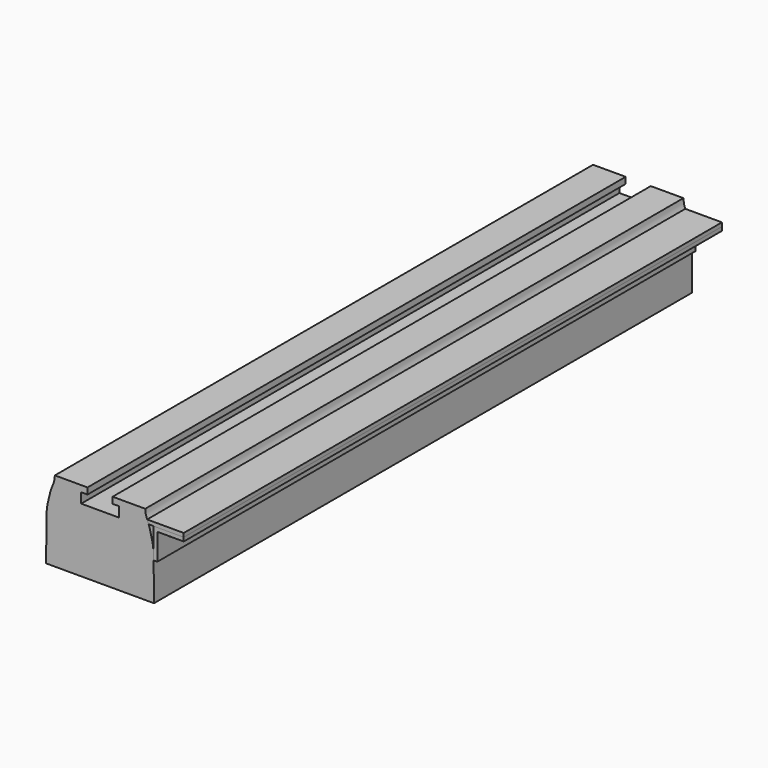
from build123d import *

# Parameters (mm, degrees)
F1_DEPTH    = 1701.8
F2_T        = 12.7
F2_T3_DEPTH = 1727.2
F3_DEPTH    = 1701.8
F4_DEPTH    = 1701.8
F5_R        = 4.7625
F6_DEPTH    = 76.2
F7_R        = 4.7625
F8_DEPTH    = 38.1
F9_DEPTH    = 7.9502


# Not quite as in the source:
# - a shell that OpenCascade refuses in one call is made with other operations: the cavity is built on its own and cut out


with BuildPart() as f1:
    # F0 (on Front) → F1 (new body)
    with BuildSketch(Plane.XZ):
        with BuildLine():
            add(Edge.make_bspline(
                [(22.225, 203.2), (21.8642991609, 198.9436880719), (21.1344297725, 190.3311442484), (16.2062788464, 177.7659442367), (11.0503834246, 165.2296560586), (8.3197375625, 152.3981513973), (4.8439366382, 139.6834435797), (2.2250256216, 127.2785692933), (1.2286177198, 113.4648940726), (1.0135363596, 99.4317737399), (0.4306333737, 42.2467726736), (0, 0)],
                knots=[0, 0, 0, 0, 0.0918377354, 0.1858314274, 0.2803034725, 0.3731848965, 0.4660441611, 0.5583399226, 0.6499464605, 0.7413896645, 1, 1, 1, 1], degree=3))
            Line((0, 0), (136.525, 0))
            Line((136.525, 0), (273.05, 0))
            add(Edge.make_bspline(
                [(272.0569275252, 95.25), (272.2812266122, 75.4195947963), (272.6656133061, 37.7097973982), (273.05, 0)],
                knots=[0.7691624061, 0.7691624061, 0.7691624061, 0.7691624061, 1, 1, 1, 1], degree=3))
            add(Edge.make_bspline(
                [(259.3917865325, 171.45), (260.1994606069, 169.3420370399), (262.4611803115, 163.060734298), (264.7302624375, 152.3981513973), (268.2060633618, 139.6834435797), (270.8249743784, 127.2785692933), (271.8213822802, 113.4648940726), (271.9240494417, 106.7663097297), (272.0299414505, 97.6358536592), (272.0569275252, 95.25)],
                knots=[0.2331960594, 0.2331960594, 0.2331960594, 0.2331960594, 0.2803034725, 0.3731848965, 0.4660441611, 0.5583399226, 0.6499464605, 0.7413896645, 0.7691624061, 0.7691624061, 0.7691624061, 0.7691624061], degree=3))
            Line((259.3917865325, 171.45), (257.0350068766, 177.3899913101))
            add(Edge.make_bspline(
                [(255.612601505, 180.975), (256.0230639926, 179.9152345168), (256.500145149, 178.7204324571), (256.980044358, 177.5266491388), (257.0350068766, 177.3899913101)],
                knots=[0.1621762876, 0.1621762876, 0.1621762876, 0.1621762876, 0.1858314274, 0.1888896754, 0.1888896754, 0.1888896754, 0.1888896754], degree=3))
            add(Edge.make_bspline(
                [(250.825, 203.2), (251.1857008391, 198.9436880719), (251.822662571, 191.4274654202), (254.3920914035, 184.1262123929), (255.612601505, 180.975)],
                knots=[0, 0, 0, 0, 0.0918377354, 0.1621762876, 0.1621762876, 0.1621762876, 0.1621762876], degree=3))
            Line((250.825, 203.2), (168.275, 203.2))
            Line((168.275, 203.2), (168.275, 187.325))
            Line((168.275, 187.325), (184.15, 187.325))
            Line((184.15, 187.325), (184.15, 161.925))
            Line((184.15, 161.925), (136.525, 161.925))
            Line((136.525, 161.925), (88.9, 161.925))
            Line((88.9, 161.925), (88.9, 187.325))
            Line((88.9, 187.325), (104.775, 187.325))
            Line((104.775, 187.325), (104.775, 203.2))
            Line((104.775, 203.2), (22.225, 203.2))
        make_face()
    extrude(amount=F1_DEPTH)

    # F2: shell of thickness 12.7, made by hand


with BuildPart() as f2_core1:
    # F2_t2: copy of F1
    add(f1.part)

    # the walls: a layer under each face that stays
    f2_faces = [f2_core1.faces().sort_by_distance(p)[0] for p in [
        (3.9234483512, -850.9, 135.090556138),
        (136.525, -1701.8, 101.6),
        (104.775, -850.9, 195.2625),
        (96.8375, -850.9, 187.325),
        (88.9, -850.9, 174.625),
        (136.525, -850.9, 161.925),
        (184.15, -850.9, 174.625),
        (176.2125, -850.9, 187.325),
        (168.275, -850.9, 195.2625),
        (209.55, -850.9, 203.2),
        (252.207010635, -850.9, 191.9731178888),
        (256.3176106399, -850.9, 179.181336214),
        (258.2133967045, -850.9, 174.4199956551),
        (269.1606720318, -850.9, 134.9300335195),
        (272.49343091, -850.9, 54.3297720729),
        (136.525, 0, 101.6),
        (63.5, -850.9, 203.2),
    ]]
    thicken(f2_faces, amount=-F2_T, mode=Mode.SUBTRACT)

    # F2_s4 → F2_t3 (cut)
    with BuildSketch(Plane.XZ.offset(-12.7)):
        Polygon((89.027, 187.198), (88.9, 200.025), (76.2, 200.025), (76.2, 187.325), align=None)
        Polygon((89.027, 162.052), (76.2, 161.925), (76.2, 149.225), (88.9, 149.225), align=None)
        Polygon((184.023, 162.052), (184.15, 149.225), (196.85, 149.225), (196.85, 161.925), align=None)
        Polygon((184.023, 187.198), (196.85, 187.325), (196.85, 200.025), (184.15, 200.025), align=None)
    extrude(amount=F2_T3_DEPTH, mode=Mode.SUBTRACT)


with BuildPart() as f1_1:
    add(f1.part)

    # what is left inside the walls is the cavity
    f2_cavity = [f2_core1.part.solids().sort_by_distance(p)[0] for p in [
        (136.525, -1130.3, 0.127),
    ]]
    add(f2_cavity, mode=Mode.SUBTRACT)


with BuildPart() as f3:
    # F0 (on Front) → F3 (new body)
    with BuildSketch(Plane.XZ):
        with BuildLine():
            add(Edge.make_bspline(
                [(257.0350068766, 177.3899913101), (257.831276655, 175.410160296), (258.6321371426, 173.4326224799), (259.3917865325, 171.45)],
                knots=[0.1888896754, 0.1888896754, 0.1888896754, 0.1888896754, 0.2331960594, 0.2331960594, 0.2331960594, 0.2331960594], degree=3))
            Line((259.3917865325, 171.45), (272.0569275252, 171.45))
            Line((272.0569275252, 171.45), (348.2569275252, 171.45))
            Line((348.2569275252, 171.45), (348.2569275252, 180.975))
            Line((348.2569275252, 180.975), (255.612601505, 180.975))
            Line((255.612601505, 180.975), (257.0350068766, 177.3899913101))
        make_face()
    extrude(amount=F3_DEPTH)


with BuildPart() as f4:
    # F0 (on Front) → F4 (new body)
    with BuildSketch(Plane.XZ):
        Polygon((272.0569275252, 171.45), (272.0569275252, 95.25), (281.5819275252, 95.25), (281.5819275252, 161.925), (348.2569275252, 161.925), (348.2569275252, 171.45), align=None)
    extrude(amount=F4_DEPTH)


with BuildPart() as f6_tool:
    # F5 (on face) → F6 (new body)
    with BuildSketch(Plane.YZ.offset(281.5819275252)):
        with Locations((-1663.7, 146.0500000011)):
            Circle(F5_R)
        with Locations((-1392.7666666667, 146.0500000011)):
            Circle(F5_R)
        with Locations((-1121.8333333333, 146.0500000011)):
            Circle(F5_R)
        with Locations((-850.9, 146.0500000011)):
            Circle(F5_R)
        with Locations((-579.9666666667, 146.0500000011)):
            Circle(F5_R)
        with Locations((-309.0333333333, 146.0500000011)):
            Circle(F5_R)
        with Locations((-38.1, 146.0500000011)):
            Circle(F5_R)
    extrude(amount=-F6_DEPTH)


with BuildPart() as f1_2:
    add(f1_1.part)

    # F6: cut by f6_tool
    add(f6_tool.part, mode=Mode.SUBTRACT)


with BuildPart() as f4_1:
    add(f4.part)

    # F6: cut by f6_tool
    add(f6_tool.part, mode=Mode.SUBTRACT)


with BuildPart() as f8:
    # F7 (on face) → F8 (new body)
    with BuildSketch(Plane.YZ.offset(281.5819275252)):
        with Locations((-1663.7, 146.0500000011)):
            Circle(F7_R)
    extrude(amount=-F8_DEPTH)

    # F7 (on face) + F5 (on face) → F9 (join)
    with BuildSketch(Plane.YZ.offset(281.5819275252)):
        Polygon((-1667.8244459855, 138.9062500011), (-1659.5755540145, 138.9062500011), (-1655.451108029, 146.0500000011), (-1659.5755540145, 153.1937500011), (-1667.8244459855, 153.1937500011), (-1671.948891971, 146.0500000011), align=None)
        with Locations((-1663.7, 146.0500000011)):
            Circle(F7_R, mode=Mode.SUBTRACT)
    with BuildSketch(Plane.YZ.offset(281.5819275252)):
        with Locations((-1663.7, 146.0500000011)):
            Circle(F5_R)
    extrude(amount=F9_DEPTH)


with BuildPart() as f8b:
    # F7 (on face) → F8, piece 2 (new body)
    with BuildSketch(Plane.YZ.offset(281.5819275252)):
        with Locations((-1392.7666666667, 146.0500000011)):
            Circle(F7_R)
    extrude(amount=-F8_DEPTH)

    # F7 (on face) + F5 (on face) → F9, piece 2 (join)
    with BuildSketch(Plane.YZ.offset(281.5819275252)):
        Polygon((-1384.5177746956, 146.0500000011), (-1388.6422206811, 153.1937500011), (-1396.8911126522, 153.1937500011), (-1401.0155586377, 146.0500000011), (-1396.8911126522, 138.9062500011), (-1388.6422206811, 138.9062500011), align=None)
        with Locations((-1392.7666666667, 146.0500000011)):
            Circle(F7_R, mode=Mode.SUBTRACT)
    with BuildSketch(Plane.YZ.offset(281.5819275252)):
        with Locations((-1392.7666666667, 146.0500000011)):
            Circle(F5_R)
    extrude(amount=F9_DEPTH)


with BuildPart() as f8c:
    # F7 (on face) → F8, piece 3 (new body)
    with BuildSketch(Plane.YZ.offset(281.5819275252)):
        with Locations((-1121.8333333333, 146.0500000011)):
            Circle(F7_R)
    extrude(amount=-F8_DEPTH)

    # F7 (on face) + F5 (on face) → F9, piece 3 (join)
    with BuildSketch(Plane.YZ.offset(281.5819275252)):
        Polygon((-1113.5844413623, 146.0500000011), (-1117.7088873478, 153.1937500011), (-1125.9577793189, 153.1937500011), (-1130.0822253044, 146.0500000011), (-1125.9577793189, 138.9062500011), (-1117.7088873478, 138.9062500011), align=None)
        with Locations((-1121.8333333333, 146.0500000011)):
            Circle(F7_R, mode=Mode.SUBTRACT)
    with BuildSketch(Plane.YZ.offset(281.5819275252)):
        with Locations((-1121.8333333333, 146.0500000011)):
            Circle(F5_R)
    extrude(amount=F9_DEPTH)


with BuildPart() as f8d:
    # F7 (on face) → F8, piece 4 (new body)
    with BuildSketch(Plane.YZ.offset(281.5819275252)):
        with Locations((-850.9, 146.0500000011)):
            Circle(F7_R)
    extrude(amount=-F8_DEPTH)

    # F7 (on face) + F5 (on face) → F9, piece 4 (join)
    with BuildSketch(Plane.YZ.offset(281.5819275252)):
        Polygon((-842.651108029, 146.0500000011), (-846.7755540145, 153.1937500011), (-855.0244459855, 153.1937500011), (-859.148891971, 146.0500000011), (-855.0244459855, 138.9062500011), (-846.7755540145, 138.9062500011), align=None)
        with Locations((-850.9, 146.0500000011)):
            Circle(F7_R, mode=Mode.SUBTRACT)
    with BuildSketch(Plane.YZ.offset(281.5819275252)):
        with Locations((-850.9, 146.0500000011)):
            Circle(F5_R)
    extrude(amount=F9_DEPTH)


with BuildPart() as f8e:
    # F7 (on face) → F8, piece 5 (new body)
    with BuildSketch(Plane.YZ.offset(281.5819275252)):
        with Locations((-579.9666666667, 146.0500000011)):
            Circle(F7_R)
    extrude(amount=-F8_DEPTH)

    # F7 (on face) + F5 (on face) → F9, piece 5 (join)
    with BuildSketch(Plane.YZ.offset(281.5819275252)):
        Polygon((-571.7177746956, 146.0500000011), (-575.8422206811, 153.1937500011), (-584.0911126522, 153.1937500011), (-588.2155586377, 146.0500000011), (-584.0911126522, 138.9062500011), (-575.8422206811, 138.9062500011), align=None)
        with Locations((-579.9666666667, 146.0500000011)):
            Circle(F7_R, mode=Mode.SUBTRACT)
    with BuildSketch(Plane.YZ.offset(281.5819275252)):
        with Locations((-579.9666666667, 146.0500000011)):
            Circle(F5_R)
    extrude(amount=F9_DEPTH)


with BuildPart() as f8f:
    # F7 (on face) → F8, piece 6 (new body)
    with BuildSketch(Plane.YZ.offset(281.5819275252)):
        with Locations((-309.0333333333, 146.0500000011)):
            Circle(F7_R)
    extrude(amount=-F8_DEPTH)

    # F7 (on face) + F5 (on face) → F9, piece 6 (join)
    with BuildSketch(Plane.YZ.offset(281.5819275252)):
        Polygon((-300.7844413623, 146.0500000011), (-304.9088873478, 153.1937500011), (-313.1577793189, 153.1937500011), (-317.2822253044, 146.0500000011), (-313.1577793189, 138.9062500011), (-304.9088873478, 138.9062500011), align=None)
        with Locations((-309.0333333333, 146.0500000011)):
            Circle(F7_R, mode=Mode.SUBTRACT)
    with BuildSketch(Plane.YZ.offset(281.5819275252)):
        with Locations((-309.0333333333, 146.0500000011)):
            Circle(F5_R)
    extrude(amount=F9_DEPTH)


with BuildPart() as f8g:
    # F7 (on face) → F8, piece 7 (new body)
    with BuildSketch(Plane.YZ.offset(281.5819275252)):
        with Locations((-38.1, 146.0500000011)):
            Circle(F7_R)
    extrude(amount=-F8_DEPTH)

    # F7 (on face) + F5 (on face) → F9, piece 7 (join)
    with BuildSketch(Plane.YZ.offset(281.5819275252)):
        Polygon((-29.851108029, 146.0500000011), (-33.9755540145, 153.1937500011), (-42.2244459855, 153.1937500011), (-46.348891971, 146.0500000011), (-42.2244459855, 138.9062500011), (-33.9755540145, 138.9062500011), align=None)
        with Locations((-38.1, 146.0500000011)):
            Circle(F7_R, mode=Mode.SUBTRACT)
    with BuildSketch(Plane.YZ.offset(281.5819275252)):
        with Locations((-38.1, 146.0500000011)):
            Circle(F5_R)
    extrude(amount=F9_DEPTH)


solid = Compound([f3.part, f1_2.part, f4_1.part, f8.part, f8b.part, f8c.part, f8d.part, f8e.part, f8f.part, f8g.part])
